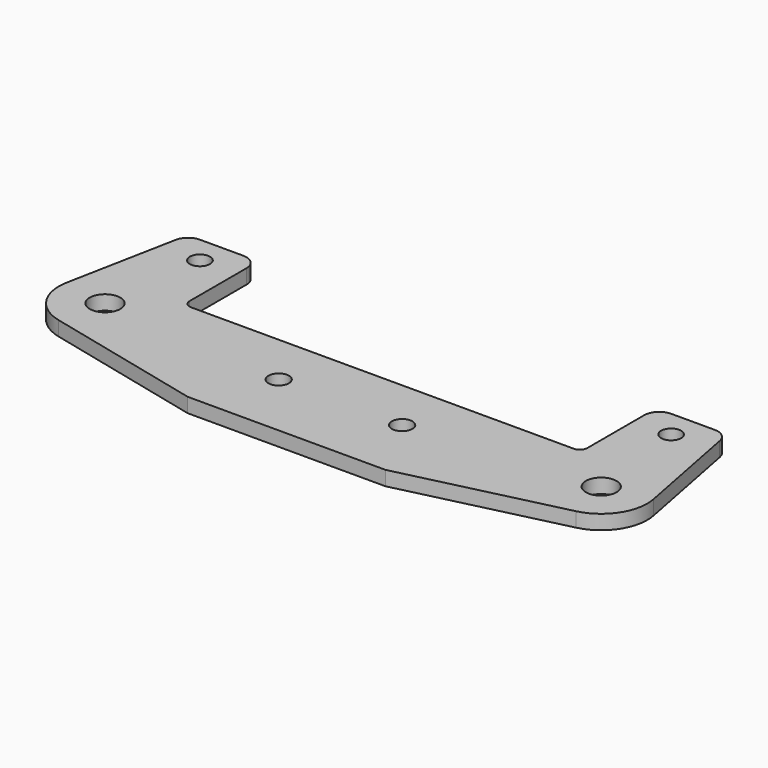
from build123d import *

# Parameters (mm, degrees)
F0_R     = 1.6706088
F0_R_2   = 1.1185144
F0_R_3   = 1.0956036
F1_DEPTH = 1.5748


# Not quite as in the source:
# - ends of sketch curves that miss each other by under 0.0002 mm in the source are joined


with BuildPart() as f1:
    # F0 (on Top) → F1 (new body)
    with BuildSketch(Plane.XY):
        with BuildLine():
            Line((-23.2852722, 11.6233956), (-25.6565654, 11.6233956))
            Line((-25.6565654, 11.6233956), (-28.0302208, 11.6233956))
            ThreePointArc((-28.0302208, 11.6233956), (-29.0641368167, 11.2522249645), (-29.6259080683, 10.3082106474))
            Line((-29.6259080683, 10.3082106474), (-31.944437, -1.6106394))
            ThreePointArc((-31.944437, -1.6106394), (-31.2390678474, -5.2827981728), (-28.1896575043, -7.446928172))
            Line((-28.1896575043, -7.446928172), (-10.768076, -11.623421))
            Line((-10.768076, -11.623421), (0, -11.623421))
            Line((0, -11.623421), (10.768076, -11.623421))
            Line((10.768076, -11.623421), (28.1896566, -7.4469244))
            ThreePointArc((28.1896566, -7.4469244), (31.2390678474, -5.2827981728), (31.9444603849, -1.610634851))
            Line((31.9444603849, -1.610634851), (29.6258996, 10.308209))
            ThreePointArc((29.6258996, 10.308209), (29.0641368167, 11.2522249645), (28.0302208, 11.6233956))
            Line((28.0302208, 11.6233956), (25.6565654, 11.6233956))
            Line((25.6565654, 11.6233956), (23.2852722, 11.6233956))
            ThreePointArc((23.2852722, 11.6233956), (22.1357994165, 11.1472683835), (21.6596722, 9.9977956))
            Line((21.6596722, 9.9977956), (21.6596722, 2.2361652))
            ThreePointArc((21.6596722, 2.2361652), (21.4216085917, 1.6614288083), (20.8468722, 1.4233652))
            Line((20.8468722, 1.4233652), (0, 1.4233652))
            Line((0, 1.4233652), (-20.8468722, 1.4233652))
            ThreePointArc((-20.8468722, 1.4233652), (-21.4216085917, 1.6614288083), (-21.6596722, 2.2361652))
            Line((-21.6596722, 2.2361652), (-21.6596722, 9.9977956))
            ThreePointArc((-21.6596722, 9.9977956), (-22.1357994165, 11.1472683835), (-23.2852722, 11.6233956))
        make_face()
        with Locations((-27.0201644, -2.5685496)):
            Circle(F0_R, mode=Mode.SUBTRACT)
        with Locations((-6.7222878, -4.3003216)):
            Circle(F0_R_2, mode=Mode.SUBTRACT)
        with Locations((6.7222878, -4.3003216)):
            Circle(F0_R_2, mode=Mode.SUBTRACT)
        with Locations((27.0201644, -2.5685496)):
            Circle(F0_R, mode=Mode.SUBTRACT)
        with Locations((-25.658445, 8.6478872)):
            Circle(F0_R_3, mode=Mode.SUBTRACT)
        with Locations((25.658445, 8.6478872)):
            Circle(F0_R_3, mode=Mode.SUBTRACT)
    extrude(amount=F1_DEPTH)


solid = f1.part
